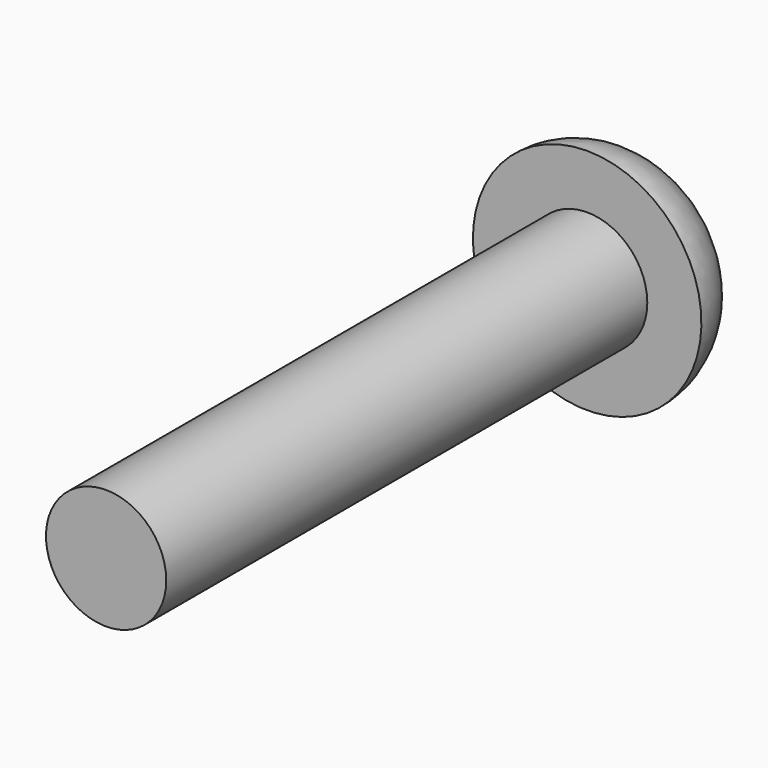
from build123d import *

# Parameters (mm, degrees)
F1_R     = 2.5
F2_DEPTH = 25
F6_DEPTH = 4


with BuildPart() as f2:
    # F1 (on Front) → F2 (new body)
    with BuildSketch(Plane.XZ):
        Circle(F1_R)
    extrude(amount=F2_DEPTH)

    # F3 (on Right) → F4 (revolve)
    with BuildSketch(Plane.YZ):
        with BuildLine():
            Line((0, 4.75), (0, 0))
            Line((0, 0), (3, 0))
            Line((3, 0), (3, 1.5))
            Line((3, 1.5), (3, 2.25))
            ThreePointArc((3, 2.25), (1.952562419, 4.0430749028), (0, 4.75))
        make_face()
    revolve(axis=Axis((0, 0, 0), (0, -1, 0)))

    # F5 (on face) → F6 (cut)
    with BuildSketch(Plane(origin=(0, 3, 0), x_dir=(-1, 0, 0), z_dir=(0, 1, 0))):
        Polygon((-1.5, 0.8660254038), (-1.5, -0.8660254038), (0, -1.7320508076), (1.5, -0.8660254038), (1.5, 0.8660254038), (0, 1.7320508076), align=None)
    extrude(amount=-F6_DEPTH, mode=Mode.SUBTRACT)


solid = f2.part
